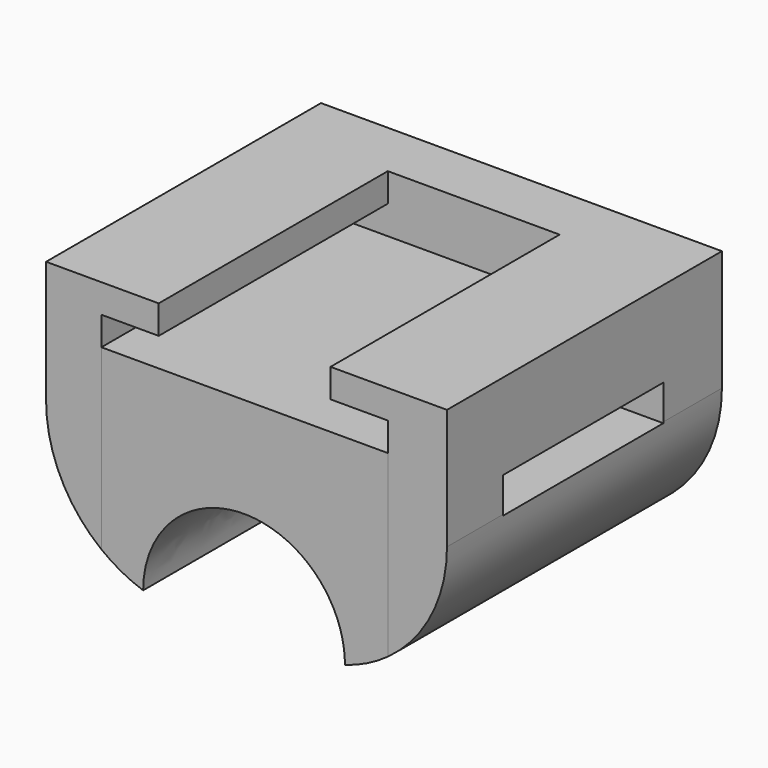
from build123d import *

# Parameters (mm, degrees)
F0_W          = 4
F0_H          = 19.9986558093
F0_W_2        = 12
F0_H_2        = 0.0013441907
F1_DEPTH      = 14
F2_DEPTH      = 18
F3_START      = 16
F3_DEPTH      = 2
F4_W          = 14
F4_H          = 2.5
F5_DEPTH      = 25
F5_DEPTH_BACK = 25
F7_DEPTH      = 25
F7_DEPTH_BACK = 25
F8_T1_DEPTH   = 71.8923030271
F8_T3_DEPTH   = 71.3347881193


# Not quite as in the source:
# - a fillet or chamfer that OpenCascade refuses, or shapes differently, is made with other operations: its cross-section is extruded or revolved along the edge and cut away or added


with BuildPart() as f1:
    # F0 (on Top) → F1 (new body)
    with BuildSketch(Plane.XY):
        Polygon((-9.9598446302, -10.1588685066), (-9.9598446302, 9.8397873028), (-5.9598446302, 9.8397873028), (6.0401553698, 9.8397873028), (10.0401553698, 9.8397873028), (10.0401553698, -10.1588685066), (14.174235519, -10.1588685066), (14.174235519, 13.8411314934), (-13.825764481, 13.8411314934), (-13.825764481, -10.1588685066), align=None)
        with Locations((-7.9598446302, -0.1595406019)):
            Rectangle(F0_W, F0_H)
        with Locations((0.0401553698, -0.1595406019)):
            Rectangle(F0_W_2, F0_H)
        with Locations((-7.9598446302, -10.1595406019)):
            Rectangle(F0_W, F0_H_2)
        with Locations((8.0401553698, -0.1595406019)):
            Rectangle(F0_W, F0_H)
        with Locations((0.0401553698, -10.1595406019)):
            Rectangle(F0_W_2, F0_H_2)
        with Locations((8.0401553698, -10.1595406019)):
            Rectangle(F0_W, F0_H_2)
    extrude(amount=F1_DEPTH)

    # F0 (on Top) → F2 (join)
    with BuildSketch(Plane.XY):
        Polygon((-9.9598446302, -10.1588685066), (-9.9598446302, 9.8397873028), (-5.9598446302, 9.8397873028), (6.0401553698, 9.8397873028), (10.0401553698, 9.8397873028), (10.0401553698, -10.1588685066), (14.174235519, -10.1588685066), (14.174235519, 13.8411314934), (-13.825764481, 13.8411314934), (-13.825764481, -10.1588685066), align=None)
    extrude(amount=F2_DEPTH)

    # F0 (on Top) → F3 (join)
    with BuildSketch(Plane.XY.offset(F3_START)):
        with Locations((8.0401553698, -0.1595406019)):
            Rectangle(F0_W, F0_H)
        with Locations((-7.9598446302, -0.1595406019)):
            Rectangle(F0_W, F0_H)
    extrude(amount=F3_DEPTH)

    # F4 (on Right) → F5 (cut, two sides)
    with BuildSketch(Plane.YZ) as f5_sk:
        with Locations((1.7279156186, 10.75)):
            Rectangle(F4_W, F4_H)
    extrude(amount=-F5_DEPTH, mode=Mode.SUBTRACT)
    extrude(f5_sk.sketch, amount=F5_DEPTH_BACK, mode=Mode.SUBTRACT)

    # F6 (on Front) → F7 (cut, two sides)
    with BuildSketch(Plane.XZ) as f7_sk:
        with BuildLine():
            add(Edge.make_bspline(
                [(7.0470551149, 0), (7.0470551149, 12.124355653), (-3.5235275575, 6.0621778265), (-14.0941102298, 0), (-3.5235275575, -6.0621778265), (7.0470551149, -12.124355653), (7.0470551149, 0)],
                knots=[0, 0, 0, 2.0943951024, 2.0943951024, 4.1887902048, 4.1887902048, 6.2831853072, 6.2831853072, 6.2831853072], degree=2, weights=[1, 0.5, 1, 0.5, 1, 0.5, 1]))
        make_face()
    extrude(amount=-F7_DEPTH, mode=Mode.SUBTRACT)
    extrude(f7_sk.sketch, amount=F7_DEPTH_BACK, mode=Mode.SUBTRACT)

    # F8: fillet of radius 10 on 2 edges, made by hand

    # F8_s2 → F8_t1 (cut)
    with BuildSketch(Plane.XZ.offset(-37.787283007)):
        with BuildLine():
            ThreePointArc((14.174235519, 9.5784606054), (12.1969593694, 3.6088792113), (7.0470551149, 0))
            Line((7.0470551149, 0), (14.174235519, 0))
            Line((14.174235519, 0), (14.174235519, 9.5784606054))
        make_face()
    extrude(amount=F8_T1_DEPTH, mode=Mode.SUBTRACT)

    # F8_s4 → F8_t3 (cut)
    with BuildSketch(Plane.XZ.offset(-37.5085255531)):
        with BuildLine():
            ThreePointArc((-13.825764481, 9.4669576239), (-11.9563519856, 3.6451411693), (-7.0470551149, 0))
            Line((-7.0470551149, 0), (-13.825764481, 0))
            Line((-13.825764481, 0), (-13.825764481, 9.4669576239))
        make_face()
    extrude(amount=F8_T3_DEPTH, mode=Mode.SUBTRACT)


solid = f1.part
